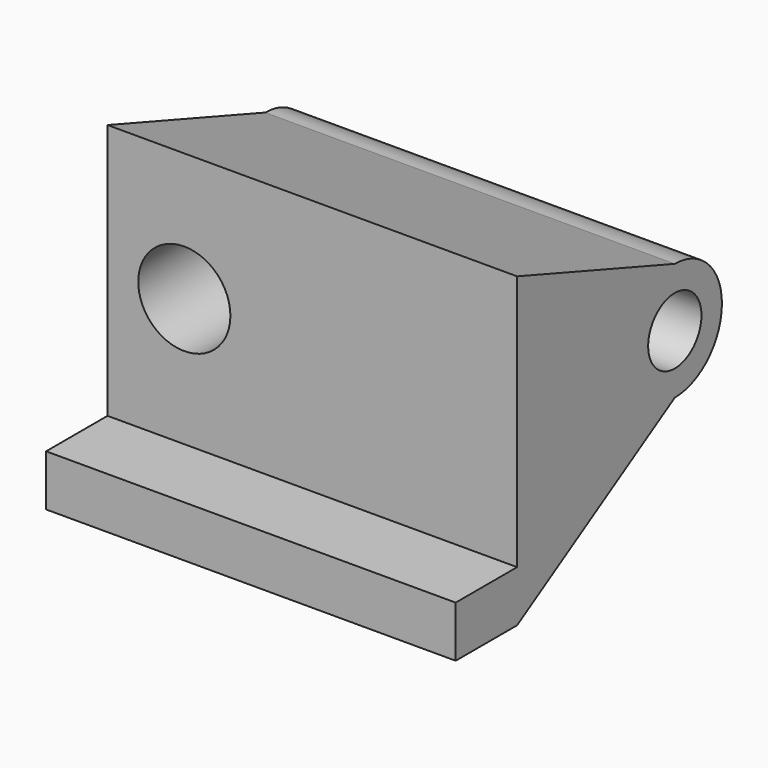
from build123d import *

# Parameters (mm, degrees)
F0_W     = 16
F0_H     = 12
F0_R     = 1.8
F1_DEPTH = 13
F2_W     = 16
F2_H     = 10
F2_R     = 1.8
F3_DEPTH = 3
F5_DEPTH = 16.001
F6_R     = 1.3
F7_DEPTH = 10


# Not quite as in the source:
# - a feature names something its author has since deleted; it is built from what else it names


with BuildPart() as f1:
    # F0 (on Front) → F1 (new body)
    with BuildSketch(Plane.XZ):
        with Locations((-5.3398377105, -1)):
            Rectangle(F0_W, F0_H)
        with Locations((-10.3398377105, 0)):
            Circle(F0_R, mode=Mode.SUBTRACT)
    extrude(amount=F1_DEPTH)

    # F2 (on face) → F3 (cut)
    with BuildSketch(Plane.XZ.offset(13)):
        with Locations((-5.3398377105, 0)):
            Rectangle(F2_W, F2_H)
        with Locations((-10.3398377105, 0)):
            Circle(F2_R, mode=Mode.SUBTRACT)
    extrude(amount=-F3_DEPTH, mode=Mode.SUBTRACT)

    # F4 (on face) → F5 (cut, through all)
    with BuildSketch(Plane.YZ.offset(2.6601622895)):
        with BuildLine():
            ThreePointArc((-2.3, 2.3), (-0.6736544033, 1.6263455967), (0, 0))
            Line((0, 0), (0, 5))
            Line((0, 5), (-10, 5))
            Line((-10, 5), (-2.3, 2.3))
        make_face()
        with BuildLine():
            Line((0, -7), (0, 0))
            ThreePointArc((0, 0), (-0.6736544033, -1.6263455967), (-2.3, -2.3))
            Line((-2.3, -2.3), (-10, -7))
            Line((-10, -7), (0, -7))
        make_face()
    extrude(amount=-F5_DEPTH, mode=Mode.SUBTRACT)

    # F6 (on face) → F7 (cut)
    with BuildSketch(Plane.YZ.offset(2.6601622895)):
        with Locations((-2.3, 0)):
            Circle(F6_R)
    extrude(amount=-F7_DEPTH, mode=Mode.SUBTRACT)


solid = f1.part
